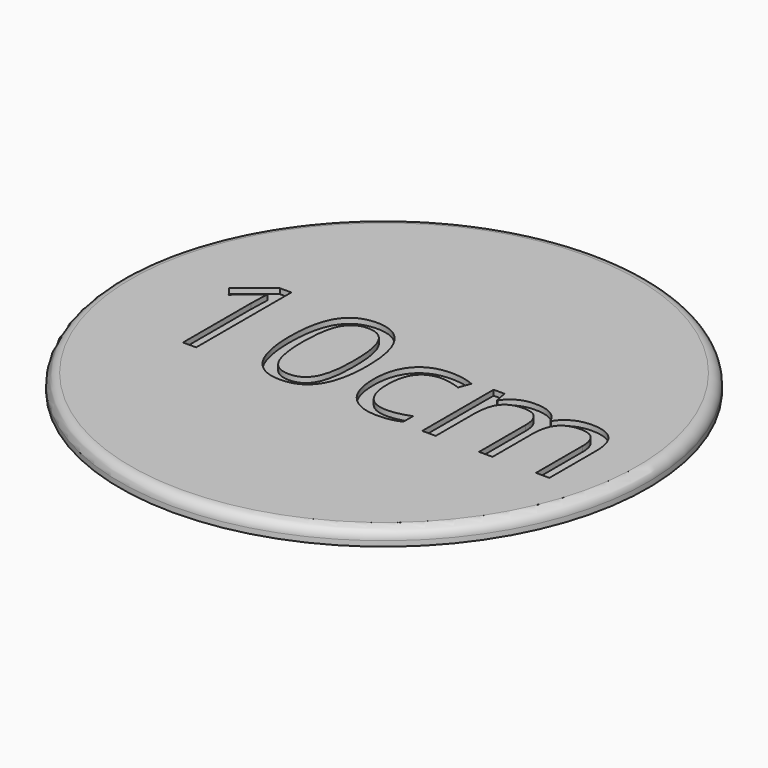
from build123d import *

# Parameters (mm, degrees)
F0_W         = 50
F0_H         = 3
F2_R         = 2
F3_TEXT_SIZE = 31.5776489454
F4_DEPTH     = 1


# Not quite as in the source:
# - Text() gives the source's letters only with a copy of the font that has no kerning and outlines rounded to 1/6400 em; it was checked with that copy


with BuildPart() as f1:
    # F0 (on Right) → F1 (revolve)
    with BuildSketch(Plane.YZ):
        with Locations((-25, 1.5)):
            Rectangle(F0_W, F0_H)
    revolve(axis=Axis((0, 0, 1.5426998725), (0, 0, 1)))

    # F2
    f2_edges = [f1.edges().sort_by_distance(p)[0] for p in [
        (0, 50, 3),
    ]]
    fillet(f2_edges, radius=F2_R)

    # F3 (on face) → F4 (cut)
    with BuildSketch(Plane.XY.offset(3)):
        with Locations((-37.7940172345, -11.031073693)):
            Text('10cm', F3_TEXT_SIZE, font='Open Sans', text_align=(TextAlign.LEFT, TextAlign.BOTTOM))
    extrude(amount=-F4_DEPTH, mode=Mode.SUBTRACT)


solid = f1.part
